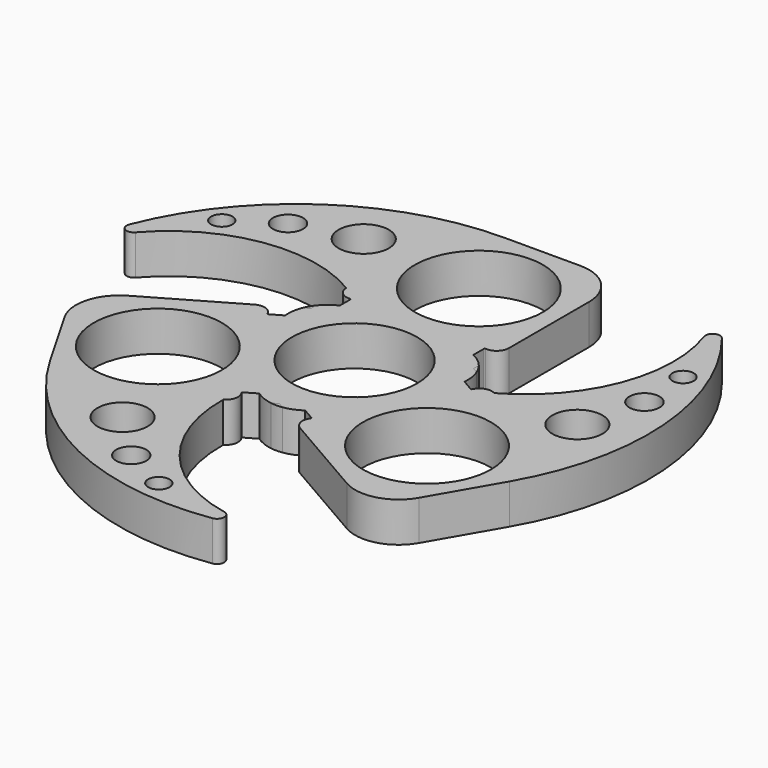
from build123d import *
from build123d import SkipClean  # not in build123d's __all__

# Parameters (mm, degrees)
F1_DEPTH  = 7
F2_DEPTH  = 33.02
F3_DEPTH  = 33.02
F4_DEPTH  = 33.02
F6_R      = 7.62
F5_R      = 11.25
F5_R_2    = 11
F7_DEPTH  = 25.4
F8_R      = 1.8749848785
F8_R_2    = 2.6443594024
F8_R_3    = 4.4059759684
F9_DEPTH  = 7
F10_R     = 1.27
F12_DEPTH = 25.4
F13_DEPTH = 7


with BuildPart() as f1:
    # F0 (on Top) → F1 (new body)
    with BuildSketch(Plane.XY):
        Polygon((14.2875, 8.248891971), (-14.2875, 8.248891971), (0, -16.4977839421), align=None)
    extrude(amount=F1_DEPTH)

    # F2 (add): a face of the model
    f2_faces = [f1.faces().sort_by_distance(p)[0] for p in [
        (-7.14375, -4.1244459855, 3.5),
    ]]
    extrude(f2_faces, amount=F2_DEPTH)

    # F3 (add): a face of the model
    f3_faces = [f1.faces().sort_by_distance(p)[0] for p in [
        (0, 8.248891971, 3.5),
    ]]
    extrude(f3_faces, amount=F3_DEPTH)

    # F4 (add): a face of the model
    f4_faces = [f1.faces().sort_by_distance(p)[0] for p in [
        (7.14375, -4.1244459855, 3.5),
    ]]
    extrude(f4_faces, amount=F4_DEPTH)

    # F6
    f6_edges = [f1.edges().sort_by_distance(p)[0] for p in [
        (-42.883659, -8.261108, 3.5),
        (-28.596159, -33.007784, 3.5),
        (28.596159, -33.007784, 3.5),
        (42.883659, -8.261108, 3.5),
        (14.2875, 41.268892, 3.5),
        (-14.2875, 41.268892, 3.5),
    ]]
    fillet(f6_edges, radius=F6_R)

    # F5 (on face) → F7 (cut)
    with BuildSketch(Plane.XY.offset(7)):
        with Locations((0, 27.298891971)):
            Circle(F5_R)
        Circle(F5_R_2)
        with BuildLine():
            ThreePointArc((34.8915339421, -13.6494459855), (12.7748683963, -10.7377317281), (33.3843197347, -19.2744459855))
            ThreePointArc((33.3843197347, -19.2744459855), (34.5081994878, -16.5611602429), (34.8915339421, -13.6494459855))
        make_face()
        with BuildLine():
            ThreePointArc((-12.3915339421, -13.6494459855), (-26.5532481995, -2.7827804398), (-33.3843197347, -19.2744459855))
            ThreePointArc((-33.3843197347, -19.2744459855), (-20.7298196847, -24.5161115313), (-12.3915339421, -13.6494459855))
        make_face()
    extrude(amount=-F7_DEPTH, mode=Mode.SUBTRACT)

    # F8 (on face) → F9 (join)
    with BuildSketch(Plane.XY.offset(7)):
        with BuildLine():
            ThreePointArc((-14.2875, 33.648891971), (-12.0556536726, 39.0370456437), (-6.6675, 41.268891971))
            ThreePointArc((-6.6675, 41.268891971), (-36.1939537613, 30.4970950948), (-51.8477511168, 3.2427063104))
            ThreePointArc((-51.8477511168, 3.2427063104), (-36.0457855424, 18.3806746008), (-14.2875, 16.048891971))
            Line((-14.2875, 16.048891971), (-14.2875, 33.648891971))
        make_face()
        with Locations((-40.1606029761, 21.0467017921)):
            Circle(F8_R, mode=Mode.SUBTRACT)
        with Locations((-32.5204535481, 26.0352350988)):
            Circle(F8_R_2, mode=Mode.SUBTRACT)
        with Locations((-21.5195283201, 28.9126522448)):
            Circle(F8_R_3, mode=Mode.SUBTRACT)
        with BuildLine():
            ThreePointArc((23.1156095166, -46.5228227514), (2.1047616282, -40.4069032795), (-6.7549981495, -20.3977839421))
            Line((-6.7549981495, -20.3977839421), (-21.9970452561, -29.1977839421))
            ThreePointArc((-21.9970452561, -29.1977839421), (-27.7792463798, -29.9590251616), (-32.406158833, -26.4086703653))
            ThreePointArc((-32.406158833, -26.4086703653), (-8.3142822131, -46.5934309681), (23.1156095166, -46.5228227514))
        make_face()
        with Locations((-6.286948215, -41.1811564646)):
            Circle(F8_R_2, mode=Mode.SUBTRACT)
        with Locations((-14.2793271748, -33.092784325)):
            Circle(F8_R_3, mode=Mode.SUBTRACT)
        with Locations((1.8533230702, -45.3034533047)):
            Circle(F8_R, mode=Mode.SUBTRACT)
        with BuildLine():
            Line((21.0424981495, 4.348891971), (21.3499965498, 4.1713576869))
            Line((21.3499965498, 4.1713576869), (36.2845452561, -4.451108029))
            ThreePointArc((36.2845452561, -4.451108029), (39.8349000524, -9.0780204821), (39.073658833, -14.8602216058))
            ThreePointArc((39.073658833, -14.8602216058), (44.5082359744, 16.0963358733), (28.7321416002, 43.280116441))
            ThreePointArc((28.7321416002, 43.280116441), (33.9410239142, 22.0262286786), (21.0424981495, 4.348891971))
        make_face()
        with Locations((35.7988554948, 4.1801320802)):
            Circle(F8_R_3, mode=Mode.SUBTRACT)
        with Locations((38.8074017631, 15.1459213658)):
            Circle(F8_R_2, mode=Mode.SUBTRACT)
        with Locations((38.3072799059, 24.2567515126)):
            Circle(F8_R, mode=Mode.SUBTRACT)
    extrude(amount=-F9_DEPTH)

    # F10
    f10_edges = [f1.edges().sort_by_distance(p)[0] for p in [
        (28.732142, 43.280116, 3.5),
        (23.11561, -46.522823, 3.5),
        (-51.847751, 3.242706, 3.5),
    ]]
    fillet(f10_edges, radius=F10_R)

    # F11 (on face) → F12 (cut)
    with BuildSketch(Plane.XY.offset(7)):
        with BuildLine():
            ThreePointArc((-15.7584187023, 4.4480611953), (-15.7224513331, 6.0815584331), (-15.3052551523, 7.6612907599))
            Line((-15.3052551523, 7.6612907599), (-21.0424981495, 4.348891971))
            ThreePointArc((-21.0424981495, 4.348891971), (-19.2958492313, 4.5353251977), (-17.9847825572, 3.3662897117))
            ThreePointArc((-17.9847825572, 3.3662897117), (-17.8870097802, 3.2797249828), (-17.7572116819, 3.2940575304))
            Line((-17.7572116819, 3.2940575304), (-15.7584187023, 4.4480611953))
        make_face()
        with BuildLine():
            ThreePointArc((-11.9076836854, 13.8921337202), (-13.5756314513, 14.443033023), (-14.2875, 16.048891971))
            Line((-14.2875, 16.048891971), (-14.2875, 9.4240943934))
            ThreePointArc((-14.2875, 9.4240943934), (-13.1280097642, 10.5752630477), (-11.7313433439, 11.423160322))
            Line((-11.7313433439, 11.423160322), (-11.7313433439, 13.7311676517))
            ThreePointArc((-11.7313433439, 13.7311676517), (-11.7838300426, 13.850742376), (-11.9076836854, 13.8921337202))
        make_face()
        with BuildLine():
            ThreePointArc((-6.0770988718, -17.2584234319), (-5.72021778, -18.9783582208), (-6.7549981495, -20.3977839421))
            Line((-6.7549981495, -20.3977839421), (-1.0177551523, -17.0853851533))
            ThreePointArc((-1.0177551523, -17.0853851533), (-2.5944415689, -16.6568214807), (-4.0270753584, -15.8712215173))
            Line((-4.0270753584, -15.8712215173), (-6.0258683381, -17.0252251822))
            ThreePointArc((-6.0258683381, -17.0252251822), (-6.1031797376, -17.1304673587), (-6.0770988718, -17.2584234319))
        make_face()
        with BuildLine():
            ThreePointArc((4.0270753584, -15.8712215173), (2.5944415689, -16.6568214807), (1.0177551523, -17.0853851533))
            Line((1.0177551523, -17.0853851533), (6.7549981495, -20.3977839421))
            ThreePointArc((6.7549981495, -20.3977839421), (5.72021778, -18.9783582208), (6.0770988718, -17.2584234319))
            ThreePointArc((6.0770988718, -17.2584234319), (6.1031797376, -17.1304673587), (6.0258683381, -17.0252251822))
            Line((6.0258683381, -17.0252251822), (4.0270753584, -15.8712215173))
        make_face()
        with BuildLine():
            Line((21.0424981495, 4.348891971), (15.3052551523, 7.6612907599))
            ThreePointArc((15.3052551523, 7.6612907599), (15.7224513331, 6.0815584331), (15.7584187023, 4.4480611953))
            Line((15.7584187023, 4.4480611953), (17.7572116819, 3.2940575304))
            ThreePointArc((17.7572116819, 3.2940575304), (17.8870097802, 3.2797249828), (17.9847825572, 3.3662897117))
            ThreePointArc((17.9847825572, 3.3662897117), (19.2958492313, 4.5353251977), (21.0424981495, 4.348891971))
        make_face()
        with BuildLine():
            Line((14.2875, 9.4240943934), (14.2875, 16.048891971))
            ThreePointArc((14.2875, 16.048891971), (13.5756314513, 14.443033023), (11.9076836854, 13.8921337202))
            ThreePointArc((11.9076836854, 13.8921337202), (11.7838300426, 13.850742376), (11.7313433439, 13.7311676517))
            Line((11.7313433439, 13.7311676517), (11.7313433439, 11.423160322))
            ThreePointArc((11.7313433439, 11.423160322), (13.1280097642, 10.5752630477), (14.2875, 9.4240943934))
        make_face()
    extrude(amount=-F12_DEPTH, mode=Mode.SUBTRACT)

    # F11 (on face) → F13 (join)
    with BuildSketch(Plane.XY.offset(7)):
        with BuildLine():
            Line((-14.2875, 8.248891971), (-14.2875, 9.4240943934))
            ThreePointArc((-14.2875, 9.4240943934), (-14.8614145652, 8.5802416998), (-15.3052551523, 7.6612907599))
            Line((-15.3052551523, 7.6612907599), (-14.2875, 8.248891971))
        make_face()
        with BuildLine():
            Line((0, -16.4977839421), (-1.0177551523, -17.0853851533))
            ThreePointArc((-1.0177551523, -17.0853851533), (0, -17.1604833996), (1.0177551523, -17.0853851533))
            Line((1.0177551523, -17.0853851533), (0, -16.4977839421))
        make_face()
        with BuildLine():
            ThreePointArc((15.3052551523, 7.6612907599), (14.8614145652, 8.5802416998), (14.2875, 9.4240943934))
            Line((14.2875, 9.4240943934), (14.2875, 8.248891971))
            Line((14.2875, 8.248891971), (15.3052551523, 7.6612907599))
        make_face()
    with SkipClean():  # cleaning this boolean's faces spoils the solid; the shape is the same uncleaned
        extrude(amount=-F13_DEPTH)


solid = f1.part
